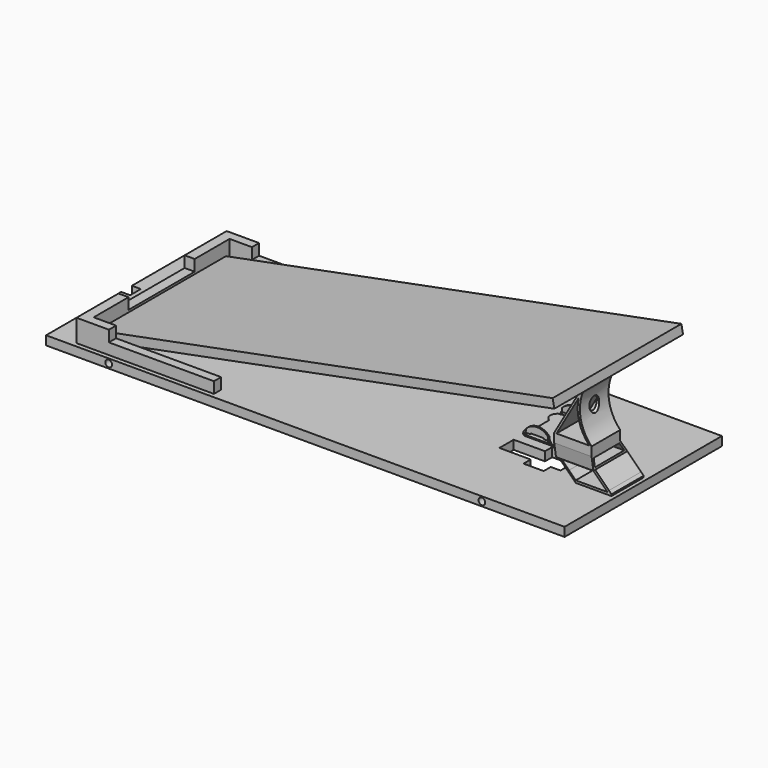
from build123d import *

# Parameters (mm, degrees)
F0_R      = 2.38125
F1_DEPTH  = 139.7
F2_W      = 6.35
F2_H      = 9.525
F3_DEPTH  = 25.4
F2_W_2    = 12.7
F2_H_2    = 31.75
F4_DEPTH  = 0.79375
F5_W      = 19.05
F5_H      = 12.7
F6_DEPTH  = 7.9375
F8_DEPTH  = 44.45
F9_W      = 11.1125
F9_H      = 9.3597000718
F10_DEPTH = 22.352
F11_DEPTH = 10.16
F12_DEPTH = 10.16
F13_DEPTH = 9.906
F14_DEPTH = 9.906
F15_DEPTH = 6.35
F2_W_3    = 38.1
F2_H_3    = 22.225
F2_H_4    = 6.35
F16_DEPTH = 12.7
F18_DEPTH = 30.48
F19_W     = 26.5225320151
F19_H     = 3.175
F19_H_2   = 28.575
F20_DEPTH = 9.525
F22_DEPTH = 31.75
F23_DEPTH = 6.35
F25_DEPTH = 25.4
F28_DEPTH = 25.4
F29_DEPTH = 127
F30_DEPTH = 12.7
F2_W_4    = 7.14375
F2_H_5    = 133.35
F31_DEPTH = 7.9375
F32_W     = 6.35
F32_H     = 7.9375
F33_DEPTH = 90.4875
F34_W     = 7.14375
F34_H     = 30.95625
F35_DEPTH = 7.9375


with BuildPart() as f1:
    # F0 (on Front) → F1 (new body)
    with BuildSketch(Plane.XZ):
        Polygon((0, -6.35), (0, 0), (-341.5624201298, 0), (-368.3, 0), (-368.3, -6.35), align=None)
        with Locations((-323.85, -3.175)):
            Circle(F0_R, mode=Mode.SUBTRACT)
        with Locations((-58.7375, -3.175)):
            Circle(F0_R, mode=Mode.SUBTRACT)
    extrude(amount=F1_DEPTH)

    # F2 (on face) → F3 (cut)
    with BuildSketch(Plane.XY):
        with Locations((-365.125, -68.2625)):
            Rectangle(F2_W, F2_H)
    extrude(amount=-F3_DEPTH, mode=Mode.SUBTRACT)

    # F2 (on face) → F15 (cut)
    with BuildSketch(Plane.XY):
        Polygon((-87.41171875, -75.6046875), (-87.41171875, -88.3046875), (-65.18671875, -88.3046875), (-65.18671875, -94.6546875), (-50.89921875, -94.6546875), (-50.89921875, -88.3046875), (-44.0232381225, -88.3046875), (-44.0232381225, -75.6046875), (-50.89921875, -75.6046875), (-50.89921875, -69.2546875), (-65.18671875, -69.2546875), (-65.18671875, -75.6046875), align=None)
    extrude(amount=-F15_DEPTH, mode=Mode.SUBTRACT)


with BuildPart() as f4:
    # F2 (on face) → F4 (new body)
    with BuildSketch(Plane.XY):
        with BuildLine():
            Line((-82.55, -36.5125), (-85.725, -36.5125))
            ThreePointArc((-85.725, -36.5125), (-88.8651367233, -41.275), (-85.725, -46.0375))
            Line((-85.725, -46.0375), (-85.725, -58.7375))
            ThreePointArc((-85.725, -58.7375), (-88.8651367233, -63.5), (-85.725, -68.2625))
            Line((-85.725, -68.2625), (-82.55, -68.2625))
            Line((-82.55, -68.2625), (-82.55, -36.5125))
        make_face()
        with Locations((-76.2, -52.3875)):
            Rectangle(F2_W_2, F2_H_2)
        with BuildLine():
            Line((-66.675, -36.5125), (-69.85, -36.5125))
            Line((-69.85, -36.5125), (-69.85, -68.2625))
            Line((-69.85, -68.2625), (-66.675, -68.2625))
            ThreePointArc((-66.675, -68.2625), (-63.5348632767, -63.5), (-66.675, -58.7375))
            Line((-66.675, -58.7375), (-66.675, -46.0375))
            ThreePointArc((-66.675, -46.0375), (-63.5348632767, -41.275), (-66.675, -36.5125))
        make_face()
    extrude(amount=F4_DEPTH)

    # F5 (on face) → F6 (join)
    with BuildSketch(Plane.XY.offset(0.79375)):
        with Locations((-76.2, -52.3875)):
            Rectangle(F5_W, F5_H)
    extrude(amount=F6_DEPTH)

    # F7 (on face) → F8 (cut)
    with BuildSketch(Plane(origin=(0, -46.0375, 0), x_dir=(-1, 0, 0), z_dir=(0, 1, 0))):
        with BuildLine():
            Line((76.2, 8.73125), (66.675, 8.73125))
            Line((66.675, 8.73125), (66.675, 0.79375))
            Line((66.675, 0.79375), (68.2625, 3.543380657))
            Line((68.2625, 3.543380657), (68.2625, 5.130880657))
            ThreePointArc((68.2625, 5.130880657), (71.8420599575, 7.789087289), (76.2, 8.73125))
        make_face()
        with BuildLine():
            Line((85.725, 8.73125), (76.2, 8.73125))
            ThreePointArc((76.2, 8.73125), (80.5579400425, 7.789087289), (84.1375, 5.130880657))
            Line((84.1375, 5.130880657), (84.1375, 3.543380657))
            Line((84.1375, 3.543380657), (85.2749538321, 1.5732528285))
            Line((85.2749538321, 1.5732528285), (85.725, 0.79375))
            Line((85.725, 0.79375), (85.725, 8.73125))
        make_face()
        Polygon((80.565625, 3.4370383213), (76.2, 3.4370383213), (76.2, 0.79375), (84.8084564477, 0.79375), (84.5875461679, 1.1763778285), (83.6792282238, 2.749630657), (80.9625, 2.749630657), align=None)
        Polygon((76.2, 0.79375), (76.2, 3.4370383213), (71.834375, 3.4370383213), (71.4375, 2.749630657), (68.7207717762, 2.749630657), (67.5915435523, 0.79375), align=None)
    extrude(amount=-F8_DEPTH, mode=Mode.SUBTRACT)

    # F9 (on face) → F10 (cut)
    with BuildSketch(Plane.YZ.offset(-66.675)):
        with Locations((-52.3875, 5.4736000359)):
            Rectangle(F9_W, F9_H)
    extrude(amount=-F10_DEPTH, mode=Mode.SUBTRACT)

    # F11 (add): a face of the model
    f11_faces = [f4.faces().sort_by_distance(p)[0] for p in [
        (-76.2, -58.7375, 5.3038676358),
    ]]
    extrude(f11_faces, amount=F11_DEPTH)

    # F12 (add): a face of the model
    f12_faces = [f4.faces().sort_by_distance(p)[0] for p in [
        (-76.2, -46.0375, 5.3038676358),
    ]]
    extrude(f12_faces, amount=F12_DEPTH)

    # F13 (cut): a face of the model
    f13_faces = [f4.faces().sort_by_distance(p)[0] for p in [
        (-76.2, -46.83125, 5.3038676358),
    ]]
    extrude(f13_faces, amount=-F13_DEPTH, mode=Mode.SUBTRACT)

    # F14 (cut): a face of the model
    f14_faces = [f4.faces().sort_by_distance(p)[0] for p in [
        (-76.2, -57.94375, 5.3038676358),
    ]]
    extrude(f14_faces, amount=-F14_DEPTH, mode=Mode.SUBTRACT)


with BuildPart() as f16:
    # F2 (on face) → F16 (new body)
    with BuildSketch(Plane.XY):
        with Locations((-21.7982381225, -77.1921875)):
            Rectangle(F2_W_3, F2_H_3)
        with Locations((-21.7982381225, -91.4796875)):
            Rectangle(F2_W_3, F2_H_4)
    extrude(amount=F16_DEPTH)

    # F17 (on face) → F18 (cut)
    with BuildSketch(Plane.XZ.offset(94.6546875)):
        Polygon((-5.4709701376, 1.6002), (-5.6628659544, 1.7920958168), (-15.4482381225, 11.5774679849), (-38.1382061073, 11.5774679849), (-32.9107381225, 6.35), (-28.1609381225, 1.6002), (-18.4952411801, 1.6002), align=None)
        Polygon((-4.5403339392, 2.9146278319), (-2.7482381225, 1.1225320151), (-2.7482381225, 12.7), (-14.3257061073, 12.7), align=None)
        Polygon((-39.7257061073, 11.5774679849), (-40.8482381225, 12.7), (-40.8482381225, 0), (-28.1482381225, 0), (-34.4982381225, 6.35), align=None)
    extrude(amount=-F18_DEPTH, mode=Mode.SUBTRACT)

    # F19 (on face) → F20 (join)
    with BuildSketch(Plane.XY.offset(12.7)):
        with Locations((-27.5869721149, -96.2421875)):
            Rectangle(F19_W, F19_H)
        with Locations((-27.5869721149, -80.3671875)):
            Rectangle(F19_W, F19_H_2)
    extrude(amount=F20_DEPTH)

    # F21 (on face) → F22 (cut)
    with BuildSketch(Plane(origin=(-40.8482381225, 0, 0), x_dir=(0, -1, 0), z_dir=(-1, 0, 0))):
        Polygon((94.9213875, 14.3002), (95.9754875, 20.6248), (74.3493643014, 20.6248), (73.2288921988, 20.6248), (68.8003596026, 14.3002), (94.6546875, 14.3002), align=None)
        Polygon((66.0796875, 12.7), (72.7491643014, 22.225), (66.0796875, 22.225), (66.0796875, 17.4625), align=None)
        Polygon((97.8296875, 12.7), (97.8296875, 22.225), (96.2421875, 12.7), align=None)
    extrude(amount=-F22_DEPTH, mode=Mode.SUBTRACT)

    # F23 (add): a face of the model
    f23_faces = [f16.faces().sort_by_distance(p)[0] for p in [
        (-27.5869721149, -85.2894259007, 22.225),
    ]]
    extrude(f23_faces, amount=F23_DEPTH)


with BuildPart() as f25:
    # F24 (on face) → F25 (new body)
    with BuildSketch(Plane.XZ.offset(97.8296875)):
        with BuildLine():
            Line((-20.2107381225, 64.3201985412), (-40.8482381225, 28.575))
            Line((-40.8482381225, 28.575), (-39.2480381225, 28.575))
            Line((-39.2480381225, 28.575), (-23.5188438749, 55.8187635989))
            ThreePointArc((-23.5188438749, 55.8187635989), (-22.1895462685, 60.1958508869), (-20.2107381225, 64.3201985412))
        make_face()
        with BuildLine():
            Line((-18.6105381225, 64.3201985412), (-20.2107381225, 64.3201985412))
            ThreePointArc((-20.2107381225, 64.3201985412), (-22.1895462685, 60.1958508869), (-23.5188438749, 55.8187635989))
            Line((-23.5188438749, 55.8187635989), (-18.6105381225, 64.3201985412))
        make_face()
        with BuildLine():
            ThreePointArc((-23.5188438749, 55.8187635989), (-23.131028165, 41.2468775416), (-15.9259061073, 28.575))
            Line((-15.9259061073, 28.575), (-14.3257061073, 28.575))
            ThreePointArc((-14.3257061073, 28.575), (-22.4196978205, 45.7341747223), (-18.6105381225, 64.3201985412))
            Line((-18.6105381225, 64.3201985412), (-23.5188438749, 55.8187635989))
        make_face()
    extrude(amount=-F25_DEPTH)

    # F27 (on offset) → F28 (cut)
    with BuildSketch(Plane(origin=(-43.0095165484, 0, 24.8315559569), x_dir=(0, -1, 0), z_dir=(-0.8660254038, 0, 0.5))):
        with BuildLine():
            Line((85.1297016859, 34.2753071345), (85.1297016859, 25.5440571345))
            ThreePointArc((85.1297016859, 25.5440571345), (88.2166647275, 26.8227190929), (89.4953266859, 29.9096821345))
            ThreePointArc((89.4953266859, 29.9096821345), (88.2166647275, 32.9966451762), (85.1297016859, 34.2753071345))
        make_face()
        with BuildLine():
            ThreePointArc((85.1297016859, 34.2753071345), (80.7640766859, 29.9096821345), (85.1297016859, 25.5440571345))
            Line((85.1297016859, 25.5440571345), (85.1297016859, 34.2753071345))
        make_face()
    extrude(amount=-F28_DEPTH, mode=Mode.SUBTRACT)


with BuildPart() as f29:
    # F0 (on Front) → F29 (new body)
    with BuildSketch(Plane.XZ):
        Polygon((-342.7740572504, 6.2333326149), (-341.5624201298, 0), (-17.4291241554, 63.0051302733), (-18.640761276, 69.2384628882), align=None)
    extrude(amount=F29_DEPTH)

    # F30 (cut): a face of the model
    f30_faces = [f29.faces().sort_by_distance(p)[0] for p in [
        (-180.1015907029, 0, 34.6192314441),
    ]]
    extrude(f30_faces, amount=-F30_DEPTH, mode=Mode.SUBTRACT)


with BuildPart() as f31:
    # F2 (on face) → F31 (new body)
    with BuildSketch(Plane.XY):
        with Locations((-345.678125, -69.85)):
            Rectangle(F2_W_4, F2_H_5)
    extrude(amount=F31_DEPTH)

    # F32 (on face) → F33 (join)
    with BuildSketch(Plane.YZ.offset(-342.10625)):
        with Locations((-6.35, 3.96875)):
            Rectangle(F32_W, F32_H)
        with Locations((-133.35, 3.96875)):
            Rectangle(F32_W, F32_H)
    extrude(amount=F33_DEPTH)

    # F34 (on face) → F35 (join)
    with BuildSketch(Plane.XY.offset(7.9375)):
        with Locations((-345.678125, -25.003125)):
            Rectangle(F34_W, F34_H)
        Polygon((-326.23125, -3.175), (-349.25, -3.175), (-349.25, -9.525), (-342.10625, -9.525), (-326.23125, -9.525), align=None)
        with Locations((-345.678125, -114.696875)):
            Rectangle(F34_W, F34_H)
        Polygon((-342.10625, -130.175), (-349.25, -130.175), (-349.25, -136.525), (-326.23125, -136.525), (-326.23125, -130.175), align=None)
    extrude(amount=F35_DEPTH)


solid = Compound([f1.part, f4.part, f16.part, f25.part, f29.part, f31.part])
